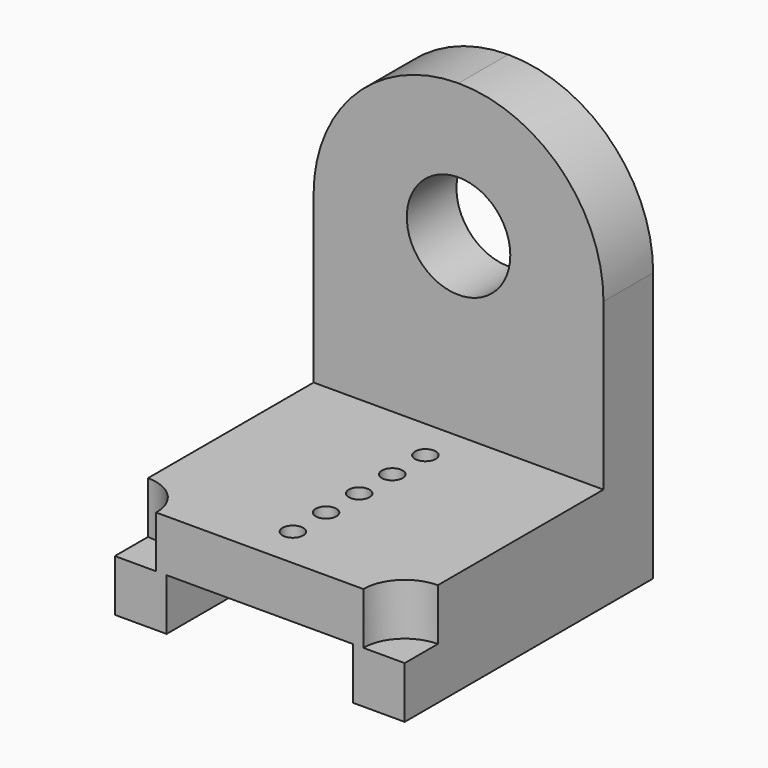
from build123d import *

# Parameters (mm, degrees)
F0_W      = 140
F0_H      = 175
F1_DEPTH  = 30
F2_R      = 69.99999
F3_R      = 25
F4_DEPTH  = 30.001
F5_W      = 140
F5_H      = 25
F6_DEPTH  = 120
F7_W      = 25
F7_H      = 150
F8_DEPTH  = 25
F9_R      = 20
F10_DEPTH = 25
F11_R     = 5
F12_DEPTH = 50.001


# Not quite as in the source:
# - a fillet or chamfer is up to 0.001 mm smaller than in the source, because OpenCascade refuses the exact size


with BuildPart() as f1:
    # F0 (on Front) → F1 (new body)
    with BuildSketch(Plane.XZ):
        Rectangle(F0_W, F0_H)
    extrude(amount=F1_DEPTH)

    # F2 (radius 70 in the source; OpenCascade refuses exactly that, so slightly less here)
    f2_edges = [f1.edges().sort_by_distance(p)[0] for p in [
        (70, -15, 87.5),
        (-70, -15, 87.5),
    ]]
    fillet(f2_edges, radius=F2_R)

    # F3 (on face) → F4 (cut, through all)
    with BuildSketch(Plane.XZ.offset(30)):
        with Locations((0, 22.5)):
            Circle(F3_R)
    extrude(amount=-F4_DEPTH, mode=Mode.SUBTRACT)

    # F5 (on face) → F6 (join)
    with BuildSketch(Plane.XZ.offset(30)):
        with Locations((0, -75)):
            Rectangle(F5_W, F5_H)
    extrude(amount=F6_DEPTH)

    # F7 (on face) → F8 (join)
    with BuildSketch(Plane(origin=(0, 0, -87.5), x_dir=(1, 0, 0), z_dir=(0, 0, -1))):
        with Locations((-57.5, 75)):
            Rectangle(F7_W, F7_H)
        with Locations((57.5, 75)):
            Rectangle(F7_W, F7_H)
    extrude(amount=F8_DEPTH)

    # F9 (on face) → F10 (cut)
    with BuildSketch(Plane.XY.offset(-62.5)):
        with Locations((-70, -150)):
            Circle(F9_R)
        with Locations((70, -150)):
            Circle(F9_R)
    extrude(amount=-F10_DEPTH, mode=Mode.SUBTRACT)

    # F11 (on face) → F12 (cut, through all)
    with BuildSketch(Plane.XY.offset(-62.5)):
        with Locations((0, -130)):
            Circle(F11_R)
        with Locations((0, -110)):
            Circle(F11_R)
        with Locations((0, -90)):
            Circle(F11_R)
        with Locations((0, -70)):
            Circle(F11_R)
        with Locations((0, -50)):
            Circle(F11_R)
    extrude(amount=-F12_DEPTH, mode=Mode.SUBTRACT)


solid = f1.part
